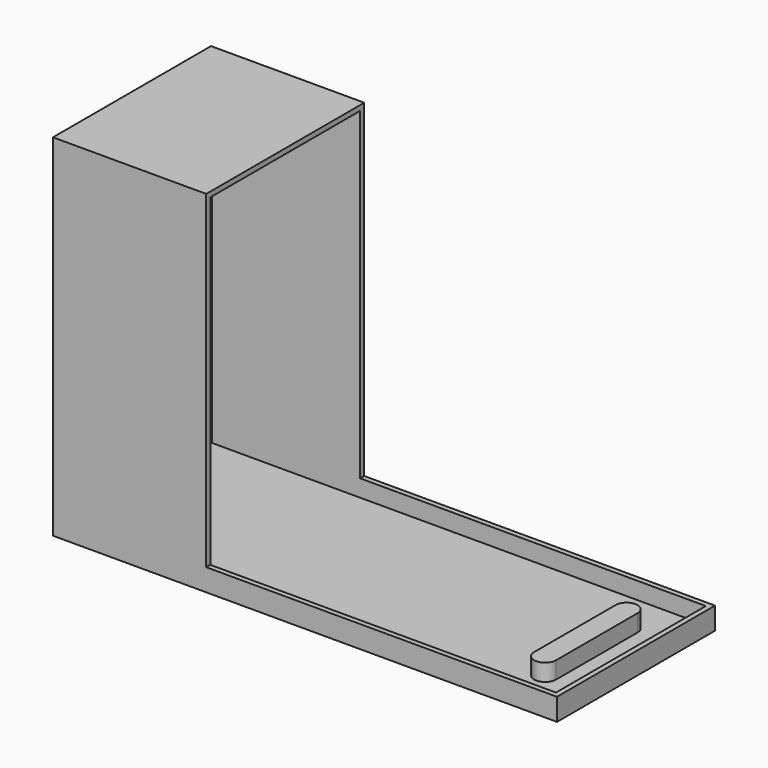
from build123d import *

# Parameters (mm, degrees)
F1_DEPTH      = 55
F1_DEPTH_BACK = 55
F4_DEPTH      = 3
F6_W          = 90
F6_H          = 116
F7_DEPTH      = 3
F9_W          = 116
F9_H          = 13
F10_DEPTH     = 3
F13_DEPTH     = 10


# Not quite as in the source:
# - a pattern or mirror of a feature is missing from the dataset's text; its kind, count and spacing are read off the source's solid


with BuildPart() as f1:
    # F0 (on Front) → F1 (new body, two sides)
    with BuildSketch(Plane.XZ) as f1_sk:
        Polygon((-49.7641339898, 203), (-49.7641339898, 0), (243.2358660102, 0), (243.2358660102, 3), (-46.7641339898, 3), (-46.7641339898, 203), align=None)
    extrude(amount=F1_DEPTH)
    extrude(f1_sk.sketch, amount=-F1_DEPTH_BACK)

    # F3 (on offset) → F4 (join)
    with BuildSketch(Plane.XZ.offset(55)):
        Polygon((40.2358660102, 203), (-49.7641339898, 203), (-49.7641339898, 0), (243.2358660102, 0), (243.2358660102, 13), (40.2358660102, 13), align=None)
    f4 = extrude(amount=F4_DEPTH)

    # F4_copies: F4 across plane
    add(f4.mirror(Plane.ZX))

    # F6 (on face) → F7 (join)
    with BuildSketch(Plane.XY.offset(203)):
        with Locations((-4.7641339898, 0)):
            Rectangle(F6_W, F6_H)
    extrude(amount=F7_DEPTH)

    # F9 (on face) → F10 (join)
    with BuildSketch(Plane.YZ.offset(243.2358660102)):
        with Locations((0, 6.5)):
            Rectangle(F9_W, F9_H)
    extrude(amount=F10_DEPTH)

    # F12 (on offset) → F13 (join)
    with BuildSketch(Plane.XY.offset(3)):
        with BuildLine():
            Line((210.3120674863, 29.9101863056), (210.3120674863, 0))
            Line((210.3120674863, 0), (210.3120674863, -29.9101863056))
            ThreePointArc((210.3120674863, -29.9101863056), (216.7739667483, -36.3720855676), (223.2358660102, -29.9101863056))
            Line((223.2358660102, -29.9101863056), (223.2358660102, 0))
            Line((223.2358660102, 0), (223.2358660102, 29.9101863056))
            ThreePointArc((223.2358660102, 29.9101863056), (216.7739667483, 36.3720855676), (210.3120674863, 29.9101863056))
        make_face()
    extrude(amount=F13_DEPTH)


solid = f1.part
